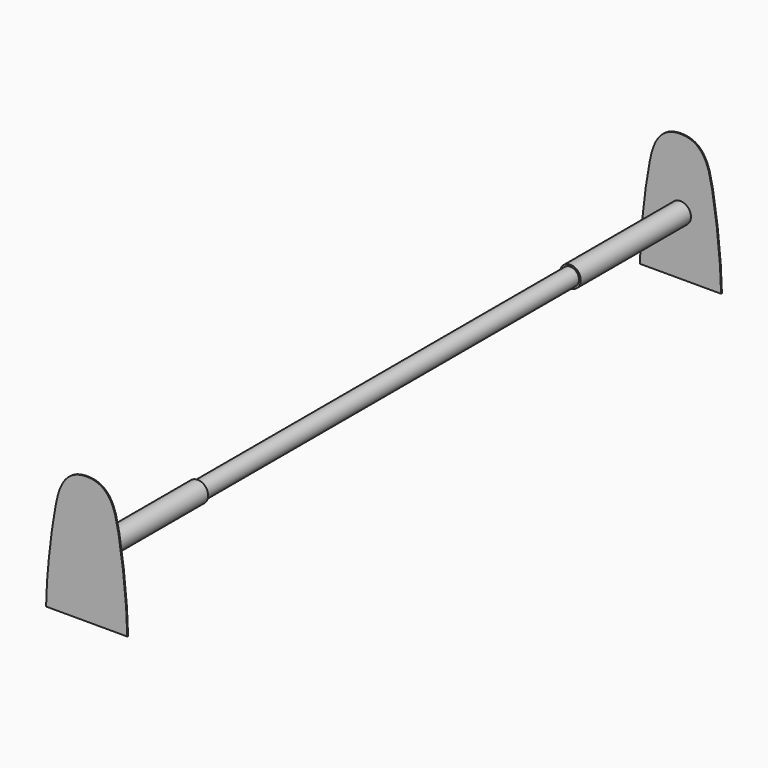
from build123d import *

# Parameters (mm, degrees)
F1_DEPTH = 2.25
F2_R     = 19.05
F2_R_2   = 16.8
F3_DEPTH = 1625.6
F5_R     = 22.86
F6_DEPTH = 301.625


# Not quite as in the source:
# - a pattern or mirror of a feature is missing from the dataset's text; its kind, count and spacing are read off the source's solid


with BuildPart() as f1:
    # F0 (on Front) → F1 (new body)
    with BuildSketch(Plane.XZ):
        with BuildLine():
            add(Edge.make_bspline(
                [(-88.9, 0), (-88.5669056837, 32.7634173245), (-82.9815055394, 99.9941611656), (-72.06314011, 188.4418096487), (-52.4019812522, 279.4), (0, 279.4)],
                knots=[0, 0, 0, 0, 0.3272882092, 0.6530732161, 1, 1, 1, 1], degree=3))
            Line((-88.9, 0), (88.9, 0))
            add(Edge.make_bspline(
                [(88.9, 0), (88.5669056837, 32.7634173245), (82.9815055394, 99.9941611656), (72.06314011, 188.4418096487), (52.4019812522, 279.4), (0, 279.4)],
                knots=[0, 0, 0, 0, 0.3272882092, 0.6530732161, 1, 1, 1, 1], degree=3))
        make_face()
    extrude(amount=-F1_DEPTH)


with BuildPart() as f1_copies_1:
    # F1_copies: instance of F1
    add(f1.part.mirror(Plane(origin=(0, -811.675, 0), x_dir=(0, 0, -1), z_dir=(0, -1, 0))))


with BuildPart() as f1_1:
    add(f1.part)

    add(f1_copies_1.part)  # F3 merges F1_copies_1
    # F2 (on face) → F3 (join)
    with BuildSketch(Plane(origin=(0, 2.25, 0), x_dir=(-1, 0, 0), z_dir=(0, 1, 0))):
        with Locations((0, 127)):
            Circle(F2_R)
        with Locations((0, 127)):
            Circle(F2_R_2, mode=Mode.SUBTRACT)
    extrude(amount=-F3_DEPTH)

    # F5 (on face) → F6 (join)
    with BuildSketch(Plane.XZ):
        with Locations((0, 127)):
            Circle(F5_R)
    f6 = extrude(amount=F6_DEPTH)

    # F6_copies: F6 across plane
    add(f6.mirror(Plane(origin=(0, -811.675, 0), x_dir=(0, 0, -1), z_dir=(0, -1, 0))))


solid = f1_1.part
